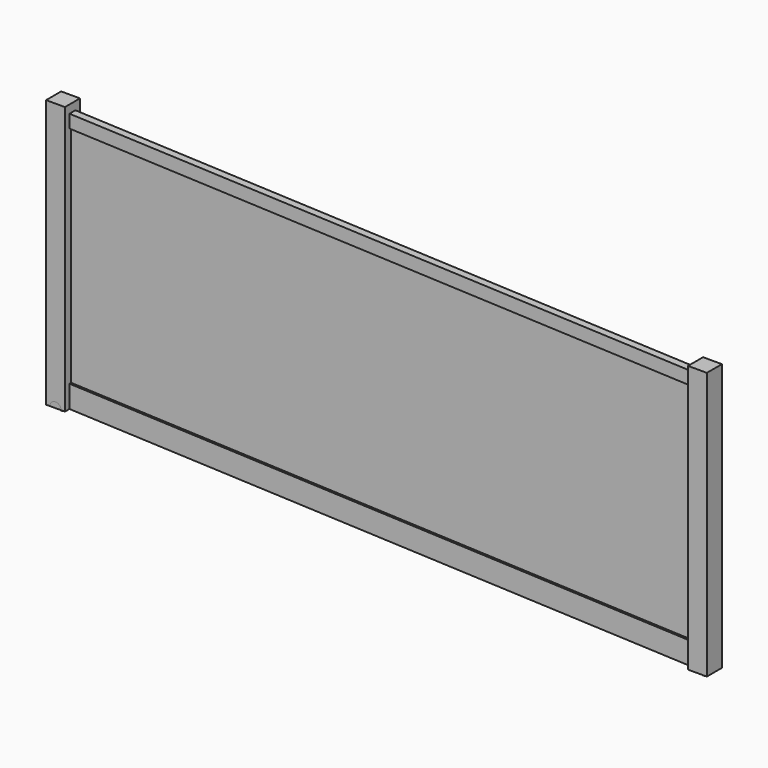
from build123d import *

# Parameters (mm, degrees)
F1_DEPTH      = 63.5
F1_DEPTH_BACK = 63.5
F2_DEPTH      = 10
F2_DEPTH_BACK = 10
F3_DEPTH      = 25
F3_DEPTH_BACK = 25
F4_DEPTH      = 11
F4_DEPTH_BACK = 11
F5_DEPTH      = 63.5
F5_DEPTH_BACK = 63.5


# Not quite as in the source:
# - a feature names something its author has since deleted; it is built from what else it names


with BuildPart() as f1:
    # F0 (on Front) → F1 (new body, two sides)
    with BuildSketch(Plane.XZ) as f1_sk:
        with BuildLine():
            Line((2142.7587509155, 1438.8117480311), (2015.7587509155, 1438.8117480311))
            Line((2015.7587509155, 1438.8117480311), (2015.7587509155, 1388.8117480311))
            Line((2015.7587509155, 1388.8117480311), (2015.7587509155, 1300.7438574954))
            Line((2015.7587509155, 1300.7438574954), (2015.7587509155, -213.5287553892))
            Line((2015.7587509155, -213.5287553892), (2015.7587509155, -363.6444778933))
            Line((2015.7587509155, -363.6444778933), (2041.7587509155, -363.6444778933))
            ThreePointArc((2041.7587509155, -363.6444778933), (2079.2587509155, -326.1444778933), (2116.7587509155, -363.6444778933))
            Line((2116.7587509155, -363.6444778933), (2142.7587509155, -363.6444778933))
            Line((2142.7587509155, -363.6444778933), (2142.7587509155, 1438.8117480311))
        make_face()
        with BuildLine():
            Line((2041.7587509155, -363.6444778933), (2116.7587509155, -363.6444778933))
            ThreePointArc((2116.7587509155, -363.6444778933), (2079.2587509155, -326.1444778933), (2041.7587509155, -363.6444778933))
        make_face()
    extrude(amount=-F1_DEPTH)
    extrude(f1_sk.sketch, amount=F1_DEPTH_BACK)


with BuildPart() as f1b:
    # F0 (on Front) → F1, piece 2 (new body, two sides)
    with BuildSketch(Plane.XZ) as f1_2_sk:
        with BuildLine():
            Line((-2285.2412490845, -198.6340780782), (-2210.2412490845, -198.6340780782))
            ThreePointArc((-2210.2412490845, -198.6340780782), (-2247.7412490845, -161.1340780782), (-2285.2412490845, -198.6340780782))
        make_face()
    extrude(amount=-F1_DEPTH)
    extrude(f1_2_sk.sketch, amount=F1_DEPTH_BACK)


with BuildPart() as f2:
    # F0 (on Front) → F2 (new body, two sides)
    with BuildSketch(Plane.XZ) as f2_sk:
        with BuildLine():
            ThreePointArc((-2285.2412490845, -198.6340780782), (-2247.7412490845, -236.1340780782), (-2210.2412490845, -198.6340780782))
            Line((-2210.2412490845, -198.6340780782), (-2285.2412490845, -198.6340780782))
        make_face()
        with BuildLine():
            Line((-2285.2412490845, -198.6340780782), (-2210.2412490845, -198.6340780782))
            ThreePointArc((-2210.2412490845, -198.6340780782), (-2247.7412490845, -161.1340780782), (-2285.2412490845, -198.6340780782))
        make_face()
    extrude(amount=F2_DEPTH)
    extrude(f2_sk.sketch, amount=-F2_DEPTH_BACK)


with BuildPart() as f2b:
    # F0 (on Front) → F2, piece 2 (new body, two sides)
    with BuildSketch(Plane.XZ) as f2_2_sk:
        with BuildLine():
            Line((2041.7587509155, -363.6444778933), (2116.7587509155, -363.6444778933))
            ThreePointArc((2116.7587509155, -363.6444778933), (2079.2587509155, -326.1444778933), (2041.7587509155, -363.6444778933))
        make_face()
        with BuildLine():
            ThreePointArc((2041.7587509155, -363.6444778933), (2079.2587509155, -401.1444778933), (2116.7587509155, -363.6444778933))
            Line((2116.7587509155, -363.6444778933), (2041.7587509155, -363.6444778933))
        make_face()
    extrude(amount=F2_DEPTH)
    extrude(f2_2_sk.sketch, amount=-F2_DEPTH_BACK)


with BuildPart() as f3:
    # F0 (on Front) → F3 (new body, two sides)
    with BuildSketch(Plane.XZ) as f3_sk:
        Polygon((2015.7587509155, -363.6444778933), (2015.7587509155, -213.5287553892), (-2184.2412490845, -48.5183555741), (-2184.2412490845, -198.6340780782), align=None)
    extrude(amount=F3_DEPTH)
    extrude(f3_sk.sketch, amount=-F3_DEPTH_BACK)


with BuildPart() as f3b:
    # F0 (on Front) → F3, piece 2 (new body, two sides)
    with BuildSketch(Plane.XZ) as f3_2_sk:
        Polygon((2015.7587509155, 1300.7438574954), (2015.7587509155, 1388.8117480311), (-2184.2412490845, 1553.8221478462), (-2184.2412490845, 1465.7542573105), align=None)
    extrude(amount=F3_DEPTH)
    extrude(f3_2_sk.sketch, amount=-F3_DEPTH_BACK)


with BuildPart() as f4:
    # F0 (on Front) → F4 (new body, two sides)
    with BuildSketch(Plane.XZ) as f4_sk:
        Polygon((2015.7587509155, -213.5287553892), (2015.7587509155, 1300.7438574954), (-2184.2412490845, 1465.7542573105), (-2184.2412490845, -48.5183555741), align=None)
    extrude(amount=F4_DEPTH)
    extrude(f4_sk.sketch, amount=-F4_DEPTH_BACK)


with BuildPart() as f5:
    # F0 (on Front) → F5 (new body, two sides)
    with BuildSketch(Plane.XZ) as f5_sk:
        with BuildLine():
            Line((-2184.2412490845, 1465.7542573105), (-2184.2412490845, 1553.8221478462))
            Line((-2184.2412490845, 1553.8221478462), (-2184.2412490845, 1603.8221478462))
            Line((-2184.2412490845, 1603.8221478462), (-2184.2412490845, 1608.8117480311))
            Line((-2184.2412490845, 1608.8117480311), (-2311.2412490845, 1608.8117480311))
            Line((-2311.2412490845, 1608.8117480311), (-2311.2412490845, -198.6340780782))
            Line((-2311.2412490845, -198.6340780782), (-2285.2412490845, -198.6340780782))
            ThreePointArc((-2285.2412490845, -198.6340780782), (-2247.7412490845, -161.1340780782), (-2210.2412490845, -198.6340780782))
            Line((-2210.2412490845, -198.6340780782), (-2184.2412490845, -198.6340780782))
            Line((-2184.2412490845, -198.6340780782), (-2184.2412490845, -48.5183555741))
            Line((-2184.2412490845, -48.5183555741), (-2184.2412490845, 1465.7542573105))
        make_face()
    extrude(amount=F5_DEPTH)
    extrude(f5_sk.sketch, amount=-F5_DEPTH_BACK)


solid = Compound([f1.part, f1b.part, f2.part, f2b.part, f3.part, f3b.part, f4.part, f5.part])
